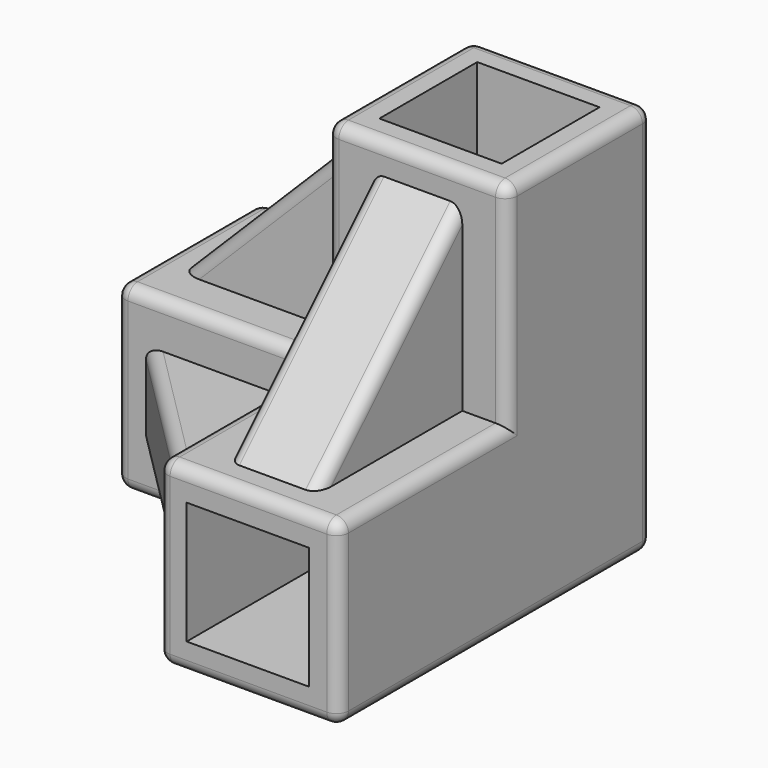
from build123d import *

# Parameters (mm, degrees)
F0_W           = 30
F0_H           = 30
F1_DEPTH       = 30
F2_W           = 30
F2_H           = 30
F2_W_2         = 20.3
F2_H_2         = 20.3
F3_DEPTH       = 35
F4_W           = 30
F4_H           = 30
F4_W_2         = 20.3
F4_H_2         = 20.3
F5_DEPTH       = 35
F6_W           = 30
F6_H           = 30
F6_W_2         = 20.3
F6_H_2         = 20.3
F7_DEPTH       = 35
F9_DEPTH       = 30
F10_W          = 7.5
F10_H          = 30
F11_DEPTH      = 35
F13_DEPTH      = 30
F15_DEPTH      = 35
F17_DEPTH      = 30
F18_W          = 35
F18_H          = 7.5
F19_DEPTH      = 35
F20_T1_DEPTH   = 26
F20_T3_DEPTH   = 26
F20_T5_DEPTH   = 33
F20_T7_DEPTH   = 33
F20_T9_DEPTH   = 26
F20_T11_DEPTH  = 33
F20_T13_DEPTH  = 61
F20_T15_DEPTH  = 61
F20_T17_DEPTH  = 33
F20_T19_DEPTH  = 33
F20_T21_DEPTH  = 33
F20_T23_DEPTH  = 61
F20_S27_W      = 2
F20_S27_H      = 2
F20_T28_DEPTH  = 2
F20_S33_W      = 2
F20_S33_H      = 2
F20_T34_DEPTH  = 2
F20_S39_W      = 2
F20_S39_H      = 2
F20_T40_DEPTH  = 2
F20_S45_W      = 2
F20_S45_H      = 2
F20_T46_DEPTH  = 2
F20_S51_W      = 2
F20_S51_H      = 2
F20_T52_DEPTH  = 2
F20_S57_W      = 2
F20_S57_H      = 2
F20_T58_DEPTH  = 2
F20_S63_W      = 2
F20_S63_H      = 2
F20_T64_DEPTH  = 2
F20_S69_W      = 2
F20_S69_H      = 2
F20_T70_DEPTH  = 2
F20_S75_W      = 2
F20_S75_H      = 2
F20_T76_DEPTH  = 2
F20_S81_W      = 2
F20_S81_H      = 2
F20_T82_DEPTH  = 2
F20_S87_W      = 2
F20_S87_H      = 2
F20_T88_DEPTH  = 2
F20_T94_DEPTH  = 52.4264068712
F20_T100_DEPTH = 52.4264068712
F20_T106_DEPTH = 52.4264068712
F20_T112_DEPTH = 52.4264068712
F20_T118_DEPTH = 52.4264068712
F20_T124_DEPTH = 52.4264068712
F20_T131_DEPTH = 38
F20_T135_DEPTH = 38
F20_T142_DEPTH = 38
F20_T146_DEPTH = 38
F20_T153_DEPTH = 38
F20_T157_DEPTH = 38
F21_T1_DEPTH   = 33
F21_T3_DEPTH   = 33
F21_S7_W       = 2
F21_S7_H       = 2
F21_T8_DEPTH   = 2
F21_S13_W      = 2
F21_S13_H      = 2
F21_T14_DEPTH  = 2
F21_T21_DEPTH  = 38
F21_S23_R      = 1.9999999999
F21_T24_DEPTH  = 21
F21_T27_DEPTH  = 38
F21_S28_R      = 1.9999999999
F21_T29_DEPTH  = 21


# Not quite as in the source:
# - a fillet or chamfer that OpenCascade refuses, or shapes differently, is made with other operations: its cross-section is extruded or revolved along the edge and cut away or added


with BuildPart() as f1:
    # F0 (on Front) → F1 (new body)
    with BuildSketch(Plane.XZ):
        with Locations((15, 15)):
            Rectangle(F0_W, F0_H)
    extrude(amount=F1_DEPTH)

    # F2 (on face) → F3 (join)
    with BuildSketch(Plane.XZ.offset(30)):
        with Locations((15, 15)):
            Rectangle(F2_W, F2_H)
        with Locations((14.9, 14.9)):
            Rectangle(F2_W_2, F2_H_2, mode=Mode.SUBTRACT)
    extrude(amount=F3_DEPTH)

    # F4 (on face) → F5 (join)
    with BuildSketch(Plane(origin=(0, 0, 0), x_dir=(0, -1, 0), z_dir=(-1, 0, 0))):
        with Locations((15, 15)):
            Rectangle(F4_W, F4_H)
        with Locations((14.9, 14.9)):
            Rectangle(F4_W_2, F4_H_2, mode=Mode.SUBTRACT)
    extrude(amount=F5_DEPTH)

    # F6 (on face) → F7 (join)
    with BuildSketch(Plane.XY.offset(30)):
        with Locations((15, -15)):
            Rectangle(F6_W, F6_H)
        with Locations((15, -15)):
            Rectangle(F6_W_2, F6_H_2, mode=Mode.SUBTRACT)
    extrude(amount=F7_DEPTH)

    # F8 (on face) → F9 (join)
    with BuildSketch(Plane.XZ.offset(30)):
        Polygon((-30, 30), (0, 30), (0, 60), align=None)
    extrude(amount=-F9_DEPTH)

    # F10 (on face) → F11 (cut)
    with BuildSketch(Plane(origin=(-35, 0, 0), x_dir=(0, -1, 0), z_dir=(-1, 0, 0))):
        with Locations((3.75, 45)):
            Rectangle(F10_W, F10_H)
        with Locations((26.25, 45)):
            Rectangle(F10_W, F10_H)
    extrude(amount=-F11_DEPTH, mode=Mode.SUBTRACT)

    # F12 (on face) → F13 (join)
    with BuildSketch(Plane(origin=(0, 0, 0), x_dir=(0, -1, 0), z_dir=(-1, 0, 0))):
        Polygon((30, 60), (30, 30), (60, 30), align=None)
    extrude(amount=-F13_DEPTH)

    # F14 (on face) → F15 (cut)
    with BuildSketch(Plane.XZ.offset(65)):
        Polygon((22.5, 60), (22.5, 30), (30, 30), (30, 65), (0, 65), (0, 30), (7.5, 30), (7.5, 60), align=None)
    extrude(amount=-F15_DEPTH, mode=Mode.SUBTRACT)

    # F16 (on face) → F17 (join)
    with BuildSketch(Plane(origin=(0, 0, 0), x_dir=(1, 0, 0), z_dir=(0, 0, -1))):
        Polygon((-30, 30), (0, 30), (0, 60), align=None)
    extrude(amount=-F17_DEPTH)

    # F18 (on face) → F19 (cut)
    with BuildSketch(Plane(origin=(-35, 0, 0), x_dir=(0, -1, 0), z_dir=(-1, 0, 0))):
        with Locations((47.5, 26.25)):
            Rectangle(F18_W, F18_H)
        with Locations((47.5, 3.75)):
            Rectangle(F18_W, F18_H)
    extrude(amount=-F19_DEPTH, mode=Mode.SUBTRACT)

    # F20: fillet of radius 2 on 28 edges, made by hand

    # F20_s2 → F20_t1 (cut)
    with BuildSketch(Plane.XZ.offset(2)):
        with BuildLine():
            ThreePointArc((-33, 30), (-34.4142135624, 29.4142135624), (-35, 28))
            Line((-35, 28), (-35, 30))
            Line((-35, 30), (-33, 30))
        make_face()
        with BuildLine():
            ThreePointArc((-35, 2), (-34.4142135624, 0.5857864376), (-33, 0))
            Line((-33, 0), (-35, 0))
            Line((-35, 0), (-35, 2))
        make_face()
        with BuildLine():
            ThreePointArc((28, 65), (29.4142135624, 64.4142135624), (30, 63))
            Line((30, 63), (30, 65))
            Line((30, 65), (28, 65))
        make_face()
    extrude(amount=F20_T1_DEPTH, mode=Mode.SUBTRACT)

    # F20_s4 → F20_t3 (cut)
    with BuildSketch(Plane.XY.offset(2)):
        with BuildLine():
            ThreePointArc((-33, -30), (-34.4142135624, -29.4142135624), (-35, -28))
            Line((-35, -28), (-35, -30))
            Line((-35, -30), (-33, -30))
        make_face()
        with BuildLine():
            ThreePointArc((-33, 0), (-34.4142135624, -0.5857864376), (-35, -2))
            Line((-35, -2), (-35, 0))
            Line((-35, 0), (-33, 0))
        make_face()
        with BuildLine():
            ThreePointArc((30, -63), (29.4142135624, -64.4142135624), (28, -65))
            Line((28, -65), (30, -65))
            Line((30, -65), (30, -63))
        make_face()
    extrude(amount=F20_T3_DEPTH, mode=Mode.SUBTRACT)

    # F20_s6 → F20_t5 (cut)
    with BuildSketch(Plane.XY.offset(2)):
        with BuildLine():
            ThreePointArc((0, -63), (0.5857864376, -64.4142135624), (2, -65))
            Line((2, -65), (0, -65))
            Line((0, -65), (0, -63))
        make_face()
    extrude(amount=F20_T5_DEPTH, mode=Mode.SUBTRACT)

    # F20_s8 → F20_t7 (cut)
    with BuildSketch(Plane.YZ.offset(-5)):
        with BuildLine():
            ThreePointArc((-65, 28), (-64.4142135624, 29.4142135624), (-63, 30))
            Line((-63, 30), (-65, 30))
            Line((-65, 30), (-65, 28))
        make_face()
        with BuildLine():
            ThreePointArc((-28, 65), (-29.4142135624, 64.4142135624), (-30, 63))
            Line((-30, 63), (-30, 65))
            Line((-30, 65), (-28, 65))
        make_face()
    extrude(amount=F20_T7_DEPTH, mode=Mode.SUBTRACT)

    # F20_s10 → F20_t9 (cut)
    with BuildSketch(Plane.YZ.offset(2)):
        with BuildLine():
            ThreePointArc((-63, 0), (-64.4142135624, 0.5857864376), (-65, 2))
            Line((-65, 2), (-65, 0))
            Line((-65, 0), (-63, 0))
        make_face()
        with BuildLine():
            ThreePointArc((-2, 65), (-0.5857864376, 64.4142135624), (0, 63))
            Line((0, 63), (0, 65))
            Line((0, 65), (-2, 65))
        make_face()
    extrude(amount=F20_T9_DEPTH, mode=Mode.SUBTRACT)

    # F20_s12 → F20_t11 (cut)
    with BuildSketch(Plane.XZ.offset(2)):
        with BuildLine():
            ThreePointArc((0, 63), (0.5857864376, 64.4142135624), (2, 65))
            Line((2, 65), (0, 65))
            Line((0, 65), (0, 63))
        make_face()
    extrude(amount=F20_T11_DEPTH, mode=Mode.SUBTRACT)

    # F20_s14 → F20_t13 (cut)
    with BuildSketch(Plane.XY.offset(2)):
        with BuildLine():
            ThreePointArc((30, -2), (29.4142135624, -0.5857864376), (28, 0))
            Line((28, 0), (30, 0))
            Line((30, 0), (30, -2))
        make_face()
    extrude(amount=F20_T13_DEPTH, mode=Mode.SUBTRACT)

    # F20_s16 → F20_t15 (cut)
    with BuildSketch(Plane.XZ.offset(2)):
        with BuildLine():
            ThreePointArc((30, 2), (29.4142135624, 0.5857864376), (28, 0))
            Line((28, 0), (30, 0))
            Line((30, 0), (30, 2))
        make_face()
    extrude(amount=F20_T15_DEPTH, mode=Mode.SUBTRACT)

    # F20_s18 → F20_t17 (cut)
    with BuildSketch(Plane.XZ.offset(30)):
        with BuildLine():
            ThreePointArc((30, 28), (29.4142135624, 29.4142135624), (28, 30))
            Line((28, 30), (30, 30))
            Line((30, 30), (30, 28))
        make_face()
        with BuildLine():
            ThreePointArc((0, 2), (0.5857864376, 0.5857864376), (2, 0))
            Line((2, 0), (0, 0))
            Line((0, 0), (0, 2))
        make_face()
    extrude(amount=F20_T17_DEPTH, mode=Mode.SUBTRACT)

    # F20_s20 → F20_t19 (cut)
    with BuildSketch(Plane.XY.offset(30)):
        with BuildLine():
            ThreePointArc((30, -28), (29.4142135624, -29.4142135624), (28, -30))
            Line((28, -30), (30, -30))
            Line((30, -30), (30, -28))
        make_face()
        with BuildLine():
            ThreePointArc((0, -2), (0.5857864376, -0.5857864376), (2, 0))
            Line((2, 0), (0, 0))
            Line((0, 0), (0, -2))
        make_face()
    extrude(amount=F20_T19_DEPTH, mode=Mode.SUBTRACT)

    # F20_s22 → F20_t21 (cut)
    with BuildSketch(Plane.YZ.offset(-33)):
        with BuildLine():
            ThreePointArc((-30, 2), (-29.4142135624, 0.5857864376), (-28, 0))
            Line((-28, 0), (-30, 0))
            Line((-30, 0), (-30, 2))
        make_face()
        with BuildLine():
            ThreePointArc((-2, 30), (-0.5857864376, 29.4142135624), (0, 28))
            Line((0, 28), (0, 30))
            Line((0, 30), (-2, 30))
        make_face()
        with BuildLine():
            ThreePointArc((-30, 28), (-29.4142135624, 29.4142135624), (-28, 30))
            Line((-28, 30), (-30, 30))
            Line((-30, 30), (-30, 28))
        make_face()
    extrude(amount=F20_T21_DEPTH, mode=Mode.SUBTRACT)

    # F20_s24 → F20_t23 (cut)
    with BuildSketch(Plane.YZ.offset(-33)):
        with BuildLine():
            ThreePointArc((0, 2), (-0.5857864376, 0.5857864376), (-2, 0))
            Line((-2, 0), (0, 0))
            Line((0, 0), (0, 2))
        make_face()
    extrude(amount=F20_T23_DEPTH, mode=Mode.SUBTRACT)


with BuildPart() as f20_tool26:
    # F20_s27 → F20_t28 (new body)
    with BuildSketch(Plane.XZ.offset(2)):
        with Locations((-34, 29)):
            Rectangle(F20_S27_W, F20_S27_H)
    extrude(amount=-F20_T28_DEPTH)

    # F20_s29 → F20_t30 (revolve, cut)
    with BuildSketch(Plane(origin=(-33, -2, 28), x_dir=(0.7071067812, 0, -0.7071067812), z_dir=(0.7071067812, 0, 0.7071067812))):
        with BuildLine():
            ThreePointArc((0, -2), (2, 0), (0, 2))
            Line((0, 2), (0, -2))
        make_face()
    revolve(axis=Axis((-33, -2, 28), (0, 1, 0)), mode=Mode.SUBTRACT)


with BuildPart() as f1_1:
    add(f1.part)

    # F20_t25: cut F20_tool26
    add(f20_tool26.part, mode=Mode.SUBTRACT)


with BuildPart() as f20_tool32:
    # F20_s33 → F20_t34 (new body)
    with BuildSketch(Plane.XZ.offset(28)):
        with Locations((-34, 29)):
            Rectangle(F20_S33_W, F20_S33_H)
    extrude(amount=F20_T34_DEPTH)

    # F20_s35 → F20_t36 (revolve, cut)
    with BuildSketch(Plane(origin=(-33, -28, 28), x_dir=(0.7071067812, 0, -0.7071067812), z_dir=(-0.7071067812, 0, -0.7071067812))):
        with BuildLine():
            ThreePointArc((0, -2), (2, 0), (0, 2))
            Line((0, 2), (0, -2))
        make_face()
    revolve(axis=Axis((-33, -28, 28), (0, -1, 0)), mode=Mode.SUBTRACT)


with BuildPart() as f1_2:
    add(f1_1.part)

    # F20_t31: cut F20_tool32
    add(f20_tool32.part, mode=Mode.SUBTRACT)


with BuildPart() as f20_tool38:
    # F20_s39 → F20_t40 (new body)
    with BuildSketch(Plane.XZ.offset(28)):
        with Locations((-34, 1)):
            Rectangle(F20_S39_W, F20_S39_H)
    extrude(amount=F20_T40_DEPTH)

    # F20_s41 → F20_t42 (revolve, cut)
    with BuildSketch(Plane(origin=(-33, -28, 2), x_dir=(0.7071067812, 0, 0.7071067812), z_dir=(0.7071067812, 0, -0.7071067812))):
        with BuildLine():
            ThreePointArc((0, -2), (2, 0), (0, 2))
            Line((0, 2), (0, -2))
        make_face()
    revolve(axis=Axis((-33, -28, 2), (0, -1, 0)), mode=Mode.SUBTRACT)


with BuildPart() as f1_3:
    add(f1_2.part)

    # F20_t37: cut F20_tool38
    add(f20_tool38.part, mode=Mode.SUBTRACT)


with BuildPart() as f20_tool44:
    # F20_s45 → F20_t46 (new body)
    with BuildSketch(Plane.XY.offset(2)):
        with Locations((-34, -1)):
            Rectangle(F20_S45_W, F20_S45_H)
    extrude(amount=-F20_T46_DEPTH)

    # F20_s47 → F20_t48 (revolve, cut)
    with BuildSketch(Plane(origin=(-33, -2, 2), x_dir=(0.7071067812, -0.7071067812, 0), z_dir=(0.7071067812, 0.7071067812, 0))):
        with BuildLine():
            ThreePointArc((0, -2), (2, 0), (0, 2))
            Line((0, 2), (0, -2))
        make_face()
    revolve(axis=Axis((-33, -2, 2), (0, 0, -1)), mode=Mode.SUBTRACT)


with BuildPart() as f1_4:
    add(f1_3.part)

    # F20_t43: cut F20_tool44
    add(f20_tool44.part, mode=Mode.SUBTRACT)


with BuildPart() as f20_tool50:
    # F20_s51 → F20_t52 (new body)
    with BuildSketch(Plane.YZ.offset(2)):
        with Locations((-64, 1)):
            Rectangle(F20_S51_W, F20_S51_H)
    extrude(amount=-F20_T52_DEPTH)

    # F20_s53 → F20_t54 (revolve, cut)
    with BuildSketch(Plane(origin=(2, -63, 2), x_dir=(0, 0.7071067812, 0.7071067812), z_dir=(0, -0.7071067812, 0.7071067812))):
        with BuildLine():
            ThreePointArc((0, -2), (2, 0), (0, 2))
            Line((0, 2), (0, -2))
        make_face()
    revolve(axis=Axis((2, -63, 2), (-1, 0, 0)), mode=Mode.SUBTRACT)


with BuildPart() as f1_5:
    add(f1_4.part)

    # F20_t49: cut F20_tool50
    add(f20_tool50.part, mode=Mode.SUBTRACT)


with BuildPart() as f20_tool56:
    # F20_s57 → F20_t58 (new body)
    with BuildSketch(Plane.YZ.offset(28)):
        with Locations((-64, 29)):
            Rectangle(F20_S57_W, F20_S57_H)
    extrude(amount=F20_T58_DEPTH)

    # F20_s59 → F20_t60 (revolve, cut)
    with BuildSketch(Plane(origin=(28, -63, 28), x_dir=(0, 0.7071067812, -0.7071067812), z_dir=(0, -0.7071067812, -0.7071067812))):
        with BuildLine():
            ThreePointArc((0, -2), (2, 0), (0, 2))
            Line((0, 2), (0, -2))
        make_face()
    revolve(axis=Axis((28, -63, 28), (1, 0, 0)), mode=Mode.SUBTRACT)


with BuildPart() as f1_6:
    add(f1_5.part)

    # F20_t55: cut F20_tool56
    add(f20_tool56.part, mode=Mode.SUBTRACT)


with BuildPart() as f20_tool62:
    # F20_s63 → F20_t64 (new body)
    with BuildSketch(Plane.YZ.offset(28)):
        with Locations((-64, 1)):
            Rectangle(F20_S63_W, F20_S63_H)
    extrude(amount=F20_T64_DEPTH)

    # F20_s65 → F20_t66 (revolve, cut)
    with BuildSketch(Plane(origin=(28, -63, 2), x_dir=(0, 0.7071067812, 0.7071067812), z_dir=(0, 0.7071067812, -0.7071067812))):
        with BuildLine():
            ThreePointArc((0, -2), (2, 0), (0, 2))
            Line((0, 2), (0, -2))
        make_face()
    revolve(axis=Axis((28, -63, 2), (1, 0, 0)), mode=Mode.SUBTRACT)


with BuildPart() as f1_7:
    add(f1_6.part)

    # F20_t61: cut F20_tool62
    add(f20_tool62.part, mode=Mode.SUBTRACT)


with BuildPart() as f20_tool68:
    # F20_s69 → F20_t70 (new body)
    with BuildSketch(Plane.YZ.offset(28)):
        with Locations((-29, 64)):
            Rectangle(F20_S69_W, F20_S69_H)
    extrude(amount=F20_T70_DEPTH)

    # F20_s71 → F20_t72 (revolve, cut)
    with BuildSketch(Plane(origin=(28, -28, 63), x_dir=(0, 0.7071067812, -0.7071067812), z_dir=(0, -0.7071067812, -0.7071067812))):
        with BuildLine():
            ThreePointArc((0, -2), (2, 0), (0, 2))
            Line((0, 2), (0, -2))
        make_face()
    revolve(axis=Axis((28, -28, 63), (1, 0, 0)), mode=Mode.SUBTRACT)


with BuildPart() as f1_8:
    add(f1_7.part)

    # F20_t67: cut F20_tool68
    add(f20_tool68.part, mode=Mode.SUBTRACT)


with BuildPart() as f20_tool74:
    # F20_s75 → F20_t76 (new body)
    with BuildSketch(Plane.YZ.offset(28)):
        with Locations((-1, 64)):
            Rectangle(F20_S75_W, F20_S75_H)
    extrude(amount=F20_T76_DEPTH)

    # F20_s77 → F20_t78 (revolve, cut)
    with BuildSketch(Plane(origin=(28, -2, 63), x_dir=(0, -0.7071067812, -0.7071067812), z_dir=(0, -0.7071067812, 0.7071067812))):
        with BuildLine():
            ThreePointArc((0, -2), (2, 0), (0, 2))
            Line((0, 2), (0, -2))
        make_face()
    revolve(axis=Axis((28, -2, 63), (1, 0, 0)), mode=Mode.SUBTRACT)


with BuildPart() as f1_9:
    add(f1_8.part)

    # F20_t73: cut F20_tool74
    add(f20_tool74.part, mode=Mode.SUBTRACT)


with BuildPart() as f20_tool80:
    # F20_s81 → F20_t82 (new body)
    with BuildSketch(Plane.YZ.offset(2)):
        with Locations((-1, 64)):
            Rectangle(F20_S81_W, F20_S81_H)
    extrude(amount=-F20_T82_DEPTH)

    # F20_s83 → F20_t84 (revolve, cut)
    with BuildSketch(Plane(origin=(2, -2, 63), x_dir=(0, -0.7071067812, -0.7071067812), z_dir=(0, 0.7071067812, -0.7071067812))):
        with BuildLine():
            ThreePointArc((0, -2), (2, 0), (0, 2))
            Line((0, 2), (0, -2))
        make_face()
    revolve(axis=Axis((2, -2, 63), (-1, 0, 0)), mode=Mode.SUBTRACT)


with BuildPart() as f1_10:
    add(f1_9.part)

    # F20_t79: cut F20_tool80
    add(f20_tool80.part, mode=Mode.SUBTRACT)


with BuildPart() as f20_tool86:
    # F20_s87 → F20_t88 (new body)
    with BuildSketch(Plane.YZ.offset(28)):
        with Locations((-1, 1)):
            Rectangle(F20_S87_W, F20_S87_H)
    extrude(amount=F20_T88_DEPTH)

    # F20_s89 → F20_t90 (revolve, cut)
    with BuildSketch(Plane(origin=(28, -2, 2), x_dir=(0, -0.7071067812, 0.7071067812), z_dir=(0, 0.7071067812, 0.7071067812))):
        with BuildLine():
            ThreePointArc((0, -2), (2, 0), (0, 2))
            Line((0, 2), (0, -2))
        make_face()
    revolve(axis=Axis((28, -2, 2), (1, 0, 0)), mode=Mode.SUBTRACT)


with BuildPart() as f1_11:
    add(f1_10.part)

    # F20_t85: cut F20_tool86
    add(f20_tool86.part, mode=Mode.SUBTRACT)


with BuildPart() as f20_tool92:
    # F20_s93 → F20_t94 (new body)
    with BuildSketch(Plane(origin=(0, -18.5355339059, -18.5355339059), x_dir=(1, 0, 0), z_dir=(0, 0.7071067812, 0.7071067812))):
        with BuildLine():
            ThreePointArc((9.5, -63.6396103068), (8.0857864376, -63.0538238692), (7.5, -61.6396103068))
            Line((7.5, -61.6396103068), (7.5, -63.6396103068))
            Line((7.5, -63.6396103068), (9.5, -63.6396103068))
        make_face()
    extrude(amount=F20_T94_DEPTH)

    split(bisect_by=Plane.XZ.offset(30), keep=Keep.TOP)

    split(bisect_by=Plane.XY.offset(30), keep=Keep.TOP)


with BuildPart() as f1_12:
    add(f1_11.part)

    # F20_t91: cut F20_tool92
    add(f20_tool92.part, mode=Mode.SUBTRACT)


with BuildPart() as f20_tool98:
    # F20_s99 → F20_t100 (new body)
    with BuildSketch(Plane(origin=(0, 18.5355339059, 18.5355339059), x_dir=(1, 0, 0), z_dir=(0, -0.7071067812, -0.7071067812))):
        with BuildLine():
            ThreePointArc((22.5, 61.6396103068), (21.9142135624, 63.0538238692), (20.5, 63.6396103068))
            Line((20.5, 63.6396103068), (22.5, 63.6396103068))
            Line((22.5, 63.6396103068), (22.5, 61.6396103068))
        make_face()
    extrude(amount=F20_T100_DEPTH)

    split(bisect_by=Plane.XZ.offset(30), keep=Keep.TOP)

    split(bisect_by=Plane.XY.offset(30), keep=Keep.TOP)


with BuildPart() as f1_13:
    add(f1_12.part)

    # F20_t97: cut F20_tool98
    add(f20_tool98.part, mode=Mode.SUBTRACT)


with BuildPart() as f20_tool104:
    # F20_s105 → F20_t106 (new body)
    with BuildSketch(Plane(origin=(33.5355339059, 0, 33.5355339059), x_dir=(0, 1, 0), z_dir=(-0.7071067812, 0, -0.7071067812))):
        with BuildLine():
            ThreePointArc((-22.5, -40.4264068712), (-21.9142135624, -41.8406204336), (-20.5, -42.4264068712))
            Line((-20.5, -42.4264068712), (-22.5, -42.4264068712))
            Line((-22.5, -42.4264068712), (-22.5, -40.4264068712))
        make_face()
    extrude(amount=F20_T106_DEPTH)

    split(bisect_by=Plane.XY.offset(30), keep=Keep.TOP)

    split(bisect_by=Plane.YZ, keep=Keep.BOTTOM)


with BuildPart() as f1_14:
    add(f1_13.part)

    # F20_t103: cut F20_tool104
    add(f20_tool104.part, mode=Mode.SUBTRACT)


with BuildPart() as f20_tool110:
    # F20_s111 → F20_t112 (new body)
    with BuildSketch(Plane(origin=(-3.5355339059, 0, -3.5355339059), x_dir=(0, 1, 0), z_dir=(0.7071067812, 0, 0.7071067812))):
        with BuildLine():
            ThreePointArc((-9.5, 42.4264068712), (-8.0857864376, 41.8406204336), (-7.5, 40.4264068712))
            Line((-7.5, 40.4264068712), (-7.5, 42.4264068712))
            Line((-7.5, 42.4264068712), (-9.5, 42.4264068712))
        make_face()
    extrude(amount=F20_T112_DEPTH)

    split(bisect_by=Plane.XY.offset(30), keep=Keep.TOP)

    split(bisect_by=Plane.YZ, keep=Keep.BOTTOM)


with BuildPart() as f1_15:
    add(f1_14.part)

    # F20_t109: cut F20_tool110
    add(f20_tool110.part, mode=Mode.SUBTRACT)


with BuildPart() as f20_tool116:
    # F20_s117 → F20_t118 (new body)
    with BuildSketch(Plane(origin=(-3.5355339059, 3.5355339059, 0), x_dir=(0, 0, 1), z_dir=(0.7071067812, -0.7071067812, 0))):
        with BuildLine():
            ThreePointArc((22.5, 40.4264068712), (21.9142135624, 41.8406204336), (20.5, 42.4264068712))
            Line((20.5, 42.4264068712), (22.5, 42.4264068712))
            Line((22.5, 42.4264068712), (22.5, 40.4264068712))
        make_face()
    extrude(amount=F20_T118_DEPTH)

    split(bisect_by=Plane.YZ, keep=Keep.BOTTOM)

    split(bisect_by=Plane.XZ.offset(30), keep=Keep.TOP)


with BuildPart() as f1_16:
    add(f1_15.part)

    # F20_t115: cut F20_tool116
    add(f20_tool116.part, mode=Mode.SUBTRACT)


with BuildPart() as f20_tool122:
    # F20_s123 → F20_t124 (new body)
    with BuildSketch(Plane(origin=(33.5355339059, -33.5355339059, 0), x_dir=(0, 0, 1), z_dir=(-0.7071067812, 0.7071067812, 0))):
        with BuildLine():
            ThreePointArc((9.5, -42.4264068712), (8.0857864376, -41.8406204336), (7.5, -40.4264068712))
            Line((7.5, -40.4264068712), (7.5, -42.4264068712))
            Line((7.5, -42.4264068712), (9.5, -42.4264068712))
        make_face()
    extrude(amount=F20_T124_DEPTH)

    split(bisect_by=Plane.YZ, keep=Keep.BOTTOM)

    split(bisect_by=Plane.XZ.offset(30), keep=Keep.TOP)


with BuildPart() as f1_17:
    add(f1_16.part)

    # F20_t121: cut F20_tool122
    add(f20_tool122.part, mode=Mode.SUBTRACT)


with BuildPart() as f20_tool129:
    # F20_s130 → F20_t131 (new body)
    with BuildSketch(Plane.XZ.offset(63)):
        with BuildLine():
            ThreePointArc((30, 28), (29.4142135624, 29.4142135624), (28, 30))
            Line((28, 30), (30, 30))
            Line((30, 30), (30, 28))
        make_face()
    extrude(amount=-F20_T131_DEPTH)

    split(bisect_by=Plane.XZ.offset(30), keep=Keep.BOTTOM)


with BuildPart() as f20_tool133:
    # F20_s134 → F20_t135 (new body)
    with BuildSketch(Plane.XY.offset(25)):
        with BuildLine():
            ThreePointArc((30, -28), (29.4142135624, -29.4142135624), (28, -30))
            Line((28, -30), (30, -30))
            Line((30, -30), (30, -28))
        make_face()
    extrude(amount=F20_T135_DEPTH)

    split(bisect_by=Plane.XY.offset(30), keep=Keep.BOTTOM)


with BuildPart() as f20_tool129_1:
    add(f20_tool129.part)

    # F20_t137: intersect F20_tool133
    add(f20_tool133.part, mode=Mode.INTERSECT)


with BuildPart() as f1_18:
    add(f1_17.part)

    # F20_t127: cut F20_tool129
    add(f20_tool129_1.part, mode=Mode.SUBTRACT)


with BuildPart() as f20_tool140:
    # F20_s141 → F20_t142 (new body)
    with BuildSketch(Plane.XZ.offset(25)):
        with BuildLine():
            ThreePointArc((0, 2), (0.5857864376, 0.5857864376), (2, 0))
            Line((2, 0), (0, 0))
            Line((0, 0), (0, 2))
        make_face()
    extrude(amount=F20_T142_DEPTH)

    split(bisect_by=Plane.XZ.offset(30), keep=Keep.BOTTOM)


with BuildPart() as f20_tool144:
    # F20_s145 → F20_t146 (new body)
    with BuildSketch(Plane.YZ.offset(-33)):
        with BuildLine():
            ThreePointArc((-30, 2), (-29.4142135624, 0.5857864376), (-28, 0))
            Line((-28, 0), (-30, 0))
            Line((-30, 0), (-30, 2))
        make_face()
    extrude(amount=F20_T146_DEPTH)

    split(bisect_by=Plane.YZ, keep=Keep.TOP)


with BuildPart() as f20_tool140_1:
    add(f20_tool140.part)

    # F20_t148: intersect F20_tool144
    add(f20_tool144.part, mode=Mode.INTERSECT)


with BuildPart() as f1_19:
    add(f1_18.part)

    # F20_t138: cut F20_tool140
    add(f20_tool140_1.part, mode=Mode.SUBTRACT)


with BuildPart() as f20_tool151:
    # F20_s152 → F20_t153 (new body)
    with BuildSketch(Plane.YZ.offset(5)):
        with BuildLine():
            ThreePointArc((-2, 30), (-0.5857864376, 29.4142135624), (0, 28))
            Line((0, 28), (0, 30))
            Line((0, 30), (-2, 30))
        make_face()
    extrude(amount=-F20_T153_DEPTH)

    split(bisect_by=Plane.YZ, keep=Keep.TOP)


with BuildPart() as f20_tool155:
    # F20_s156 → F20_t157 (new body)
    with BuildSketch(Plane.XY.offset(25)):
        with BuildLine():
            ThreePointArc((0, -2), (0.5857864376, -0.5857864376), (2, 0))
            Line((2, 0), (0, 0))
            Line((0, 0), (0, -2))
        make_face()
    extrude(amount=F20_T157_DEPTH)

    split(bisect_by=Plane.XY.offset(30), keep=Keep.BOTTOM)


with BuildPart() as f20_tool151_1:
    add(f20_tool151.part)

    # F20_t159: intersect F20_tool155
    add(f20_tool155.part, mode=Mode.INTERSECT)


with BuildPart() as f1_20:
    add(f1_19.part)

    # F20_t149: cut F20_tool151
    add(f20_tool151_1.part, mode=Mode.SUBTRACT)

    # F21: fillet of radius 2 on 2 edges, made by hand

    # F21_s2 → F21_t1 (cut)
    with BuildSketch(Plane.XY.offset(30)):
        with BuildLine():
            ThreePointArc((0, -28), (0.5857864376, -29.4142135624), (2, -30))
            Line((2, -30), (0, -30))
            Line((0, -30), (0, -28))
        make_face()
    extrude(amount=F21_T1_DEPTH, mode=Mode.SUBTRACT)

    # F21_s4 → F21_t3 (cut)
    with BuildSketch(Plane.XZ.offset(30)):
        with BuildLine():
            ThreePointArc((0, 28), (0.5857864376, 29.4142135624), (2, 30))
            Line((2, 30), (0, 30))
            Line((0, 30), (0, 28))
        make_face()
    extrude(amount=F21_T3_DEPTH, mode=Mode.SUBTRACT)


with BuildPart() as f21_tool6:
    # F21_s7 → F21_t8 (new body)
    with BuildSketch(Plane.YZ.offset(2)):
        with Locations((-64, 29)):
            Rectangle(F21_S7_W, F21_S7_H)
    extrude(amount=-F21_T8_DEPTH)

    # F21_s9 → F21_t10 (revolve, cut)
    with BuildSketch(Plane(origin=(2, -63, 28), x_dir=(0, 0.7071067812, -0.7071067812), z_dir=(0, 0.7071067812, 0.7071067812))):
        with BuildLine():
            ThreePointArc((0, -2), (2, 0), (0, 2))
            Line((0, 2), (0, -2))
        make_face()
    revolve(axis=Axis((2, -63, 28), (-1, 0, 0)), mode=Mode.SUBTRACT)


with BuildPart() as f1_21:
    add(f1_20.part)

    # F21_t5: cut F21_tool6
    add(f21_tool6.part, mode=Mode.SUBTRACT)


with BuildPart() as f21_tool12:
    # F21_s13 → F21_t14 (new body)
    with BuildSketch(Plane.YZ.offset(2)):
        with Locations((-29, 64)):
            Rectangle(F21_S13_W, F21_S13_H)
    extrude(amount=-F21_T14_DEPTH)

    # F21_s15 → F21_t16 (revolve, cut)
    with BuildSketch(Plane(origin=(2, -28, 63), x_dir=(0, 0.7071067812, -0.7071067812), z_dir=(0, 0.7071067812, 0.7071067812))):
        with BuildLine():
            ThreePointArc((0, -2), (2, 0), (0, 2))
            Line((0, 2), (0, -2))
        make_face()
    revolve(axis=Axis((2, -28, 63), (-1, 0, 0)), mode=Mode.SUBTRACT)


with BuildPart() as f1_22:
    add(f1_21.part)

    # F21_t11: cut F21_tool12
    add(f21_tool12.part, mode=Mode.SUBTRACT)


with BuildPart() as f21_tool19:
    # F21_s20 → F21_t21 (new body)
    with BuildSketch(Plane.XZ.offset(63)):
        with BuildLine():
            ThreePointArc((0, 28), (0.5857864376, 29.4142135624), (2, 30))
            Line((2, 30), (0, 30))
            Line((0, 30), (0, 28))
        make_face()
    extrude(amount=-F21_T21_DEPTH)

    split(bisect_by=Plane.XZ.offset(30), keep=Keep.BOTTOM)

    # F21_s23 → F21_t24 (cut, symmetric)
    with BuildSketch(Plane.YZ.offset(1)):
        with Locations((-28.0000000001, 28.0000000001)):
            Circle(F21_S23_R)
    extrude(amount=F21_T24_DEPTH, both=True, mode=Mode.SUBTRACT)


with BuildPart() as f21_tool25:
    # F21_s26 → F21_t27 (new body)
    with BuildSketch(Plane.XY.offset(63)):
        with BuildLine():
            ThreePointArc((0, -28), (0.5857864376, -29.4142135624), (2, -30))
            Line((2, -30), (0, -30))
            Line((0, -30), (0, -28))
        make_face()
    extrude(amount=-F21_T27_DEPTH)

    # F21_s28 → F21_t29 (cut, symmetric)
    with BuildSketch(Plane.YZ.offset(1)):
        with Locations((-28.0000000001, 28.0000000001)):
            Circle(F21_S28_R)
    extrude(amount=F21_T29_DEPTH, both=True, mode=Mode.SUBTRACT)

    split(bisect_by=Plane.XY.offset(30), keep=Keep.BOTTOM)


with BuildPart() as f21_tool19_1:
    add(f21_tool19.part)

    # F21_t31: intersect F21_tool25
    add(f21_tool25.part, mode=Mode.INTERSECT)


with BuildPart() as f1_23:
    add(f1_22.part)

    # F21_t17: cut F21_tool19
    add(f21_tool19_1.part, mode=Mode.SUBTRACT)


solid = f1_23.part
